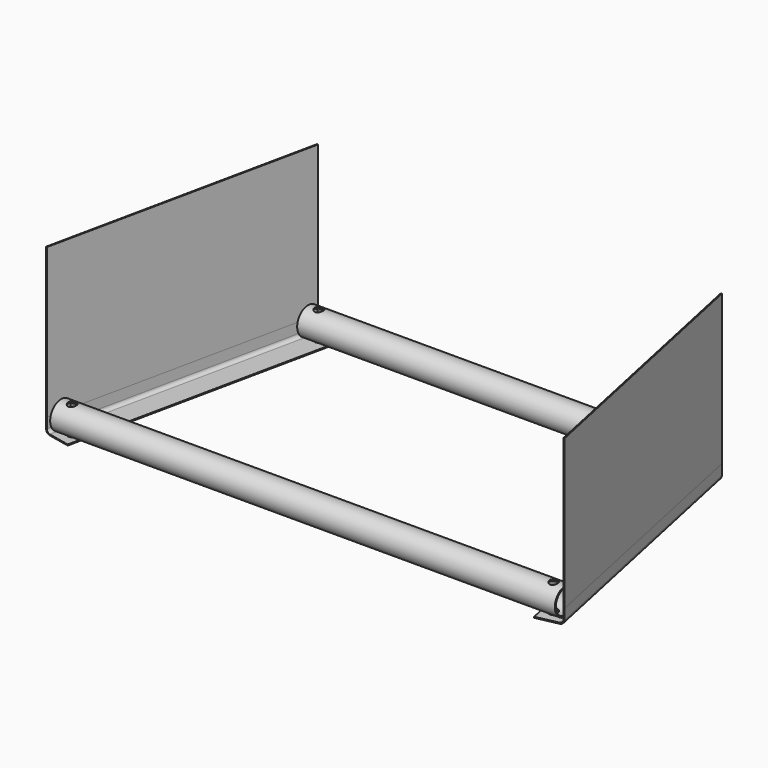
from build123d import *

# Parameters (mm, degrees)
F0_R      = 16
F0_R_2    = 14.4
F1_DEPTH  = 295
F2_R      = 16
F2_R_2    = 14.4
F3_DEPTH  = 235
F5_DEPTH  = 175
F7_DEPTH  = 320
F9_R      = 5
F10_DEPTH = 34


# Not quite as in the source:
# - a feature of the source that left no trace in its solid (it failed there, or was rolled back) is left out


with BuildPart() as f1:
    # F0 (on Right) → F1 (new body, symmetric)
    with BuildSketch(Plane.YZ):
        with Locations((-143, 0)):
            Circle(F0_R)
        with Locations((-143, 0)):
            Circle(F0_R_2, mode=Mode.SUBTRACT)
    extrude(amount=F1_DEPTH, both=True)


with BuildPart() as f3:
    # F2 (on Right) → F3 (new body, symmetric)
    with BuildSketch(Plane.YZ):
        with Locations((143, 0)):
            Circle(F2_R)
        with Locations((143, 0)):
            Circle(F2_R_2, mode=Mode.SUBTRACT)
    extrude(amount=F3_DEPTH, both=True)


with BuildPart() as f5:
    # F4 (on Top) → F5 (new body)
    with BuildSketch(Plane.XY):
        Polygon((235.4682589383, 158), (302, -155.0072322348), (303.1737771209, -154.7577382058), (236.6420360592, 158.249494029), align=None)
    extrude(amount=F5_DEPTH)

    # F6 (on face) → F7 (join)
    with BuildSketch(Plane(origin=(44.5781965418, -209.7239256768, 0), x_dir=(0.9781476007, 0.2079116908, 0), z_dir=(0.2079116908, -0.9781476007, 0))):
        with BuildLine():
            Line((264.3727596787, 0), (263.1727596787, 0))
            Line((263.1727596787, 0), (263.1727596787, -12))
            ThreePointArc((263.1727596787, -12), (262.0011868034, -14.8284271247), (259.1727596787, -16))
            Line((259.1727596787, -16), (233.1727596787, -16))
            Line((233.1727596787, -16), (233.1727596787, -17.2))
            Line((233.1727596787, -17.2), (259.3727596787, -17.2))
            ThreePointArc((259.3727596787, -17.2), (262.9082935846, -15.7355339059), (264.3727596787, -12.2))
            Line((264.3727596787, -12.2), (264.3727596787, 0))
        make_face()
    extrude(amount=-F7_DEPTH)


with BuildPart() as f8_1:
    # F8: instance of F5
    add(f5.part.mirror(Plane.YZ))


with BuildPart() as f10_tool:
    # F9 (on face) → F10 (new body)
    with BuildSketch(Plane(origin=(0, 0, -17.2), x_dir=(1, 0, 0), z_dir=(0, 0, -1))):
        with Locations((281.7637416249, 143.9734728131)):
            Circle(F9_R)
        with Locations((-281.2362583751, 143.9734728131)):
            Circle(F9_R)
        with Locations((220.8456162153, -142.6237742019)):
            Circle(F9_R)
        with Locations((-222.1543837847, -142.6237742019)):
            Circle(F9_R)
    extrude(amount=-F10_DEPTH)


with BuildPart() as f1_1:
    add(f1.part)

    # F10: cut by f10_tool
    add(f10_tool.part, mode=Mode.SUBTRACT)


with BuildPart() as f3_1:
    add(f3.part)

    # F10: cut by f10_tool
    add(f10_tool.part, mode=Mode.SUBTRACT)


with BuildPart() as f5_1:
    add(f5.part)

    # F10: cut by f10_tool
    add(f10_tool.part, mode=Mode.SUBTRACT)


with BuildPart() as f8_1_1:
    add(f8_1.part)

    # F10: cut by f10_tool
    add(f10_tool.part, mode=Mode.SUBTRACT)


solid = Compound([f1_1.part, f3_1.part, f5_1.part, f8_1_1.part])
